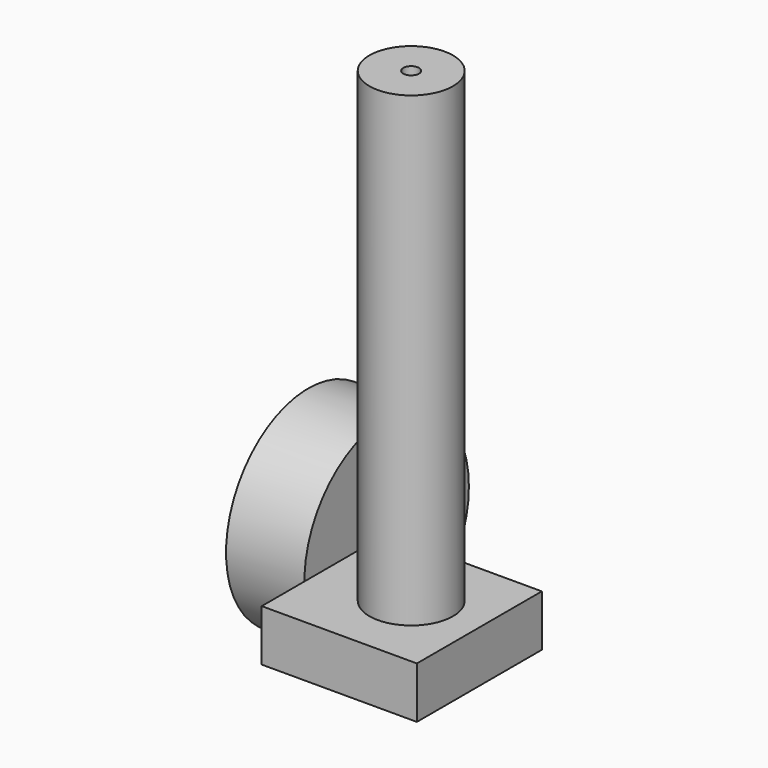
from build123d import *

# Parameters (mm, degrees)
F0_R     = 32.8057218661
F1_DEPTH = 25
F2_W     = 49.826644361
F2_H     = 16.4276733994
F3_DEPTH = 49.5127849281
F7_R     = 13.3298307558
F4_DEPTH = 148.9010583609
F8_D     = 5


# Not quite as in the source:
# - the program builds the solid bodies; features that only make, move or delete a surface that nothing else refers to are left out


with BuildPart() as f1:
    # F0 (on Right) → F1 (new body)
    with BuildSketch(Plane.YZ):
        with Locations((-28.0562192202, 48.4330356121)):
            Circle(F0_R)
    extrude(amount=F1_DEPTH)


with BuildPart() as f3:
    # F2 (on face) → F3 (new body)
    with BuildSketch(Plane.YZ.offset(25)):
        with Locations((-52.9695414007, 40.2191989124)):
            Rectangle(F2_W, F2_H)
    extrude(amount=F3_DEPTH)

    # F7 (on face) → F4 (join)
    with BuildSketch(Plane.XY.offset(48.4330356121)):
        with Locations((52.2981211543, -52.3791536689)):
            Circle(F7_R)
    extrude(amount=F4_DEPTH)

    # F8 (through all)
    with Locations(Plane.XY.offset(197.334093973)):
        with Locations((52.2981211543, -52.3791536689)):
            Hole(F8_D / 2)


solid = Compound([f1.part, f3.part])
